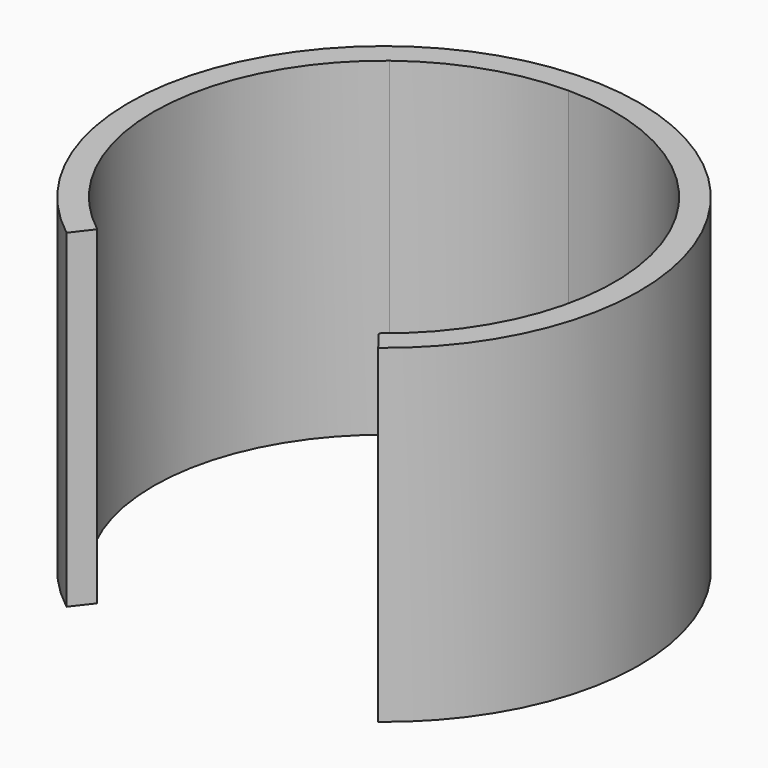
from build123d import *

# Parameters (mm, degrees)
F1_DEPTH = 200


with BuildPart() as f1:
    # F0 (on Top) → F1 (new body)
    with BuildSketch(Plane.XY):
        with BuildLine():
            ThreePointArc((0, 155), (-50, 146.7140075112), (-94.6541983943, 122.7419354839))
            ThreePointArc((-94.6541983943, 122.7419354839), (-155, 0), (-94.6541983943, -122.7419354839))
            Line((-94.6541983943, -122.7419354839), (-85.4941146788, -110.8636836629))
            ThreePointArc((-85.4941146788, -110.8636836629), (-140, 0), (-85.4941146788, 110.8636836629))
            ThreePointArc((-85.4941146788, 110.8636836629), (-45.1612903226, 132.5158777521), (0, 140))
            Line((0, 140), (0, 155))
        make_face()
        with BuildLine():
            ThreePointArc((94.6541983943, -122.7419354839), (146.7140075112, 50), (0, 155))
            Line((0, 155), (0, 140))
            ThreePointArc((0, 140), (132.5158777521, 45.1612903226), (85.4941146788, -110.8636836629))
            Line((85.4941146788, -110.8636836629), (94.6541983943, -122.7419354839))
        make_face()
    extrude(amount=F1_DEPTH)


solid = f1.part
